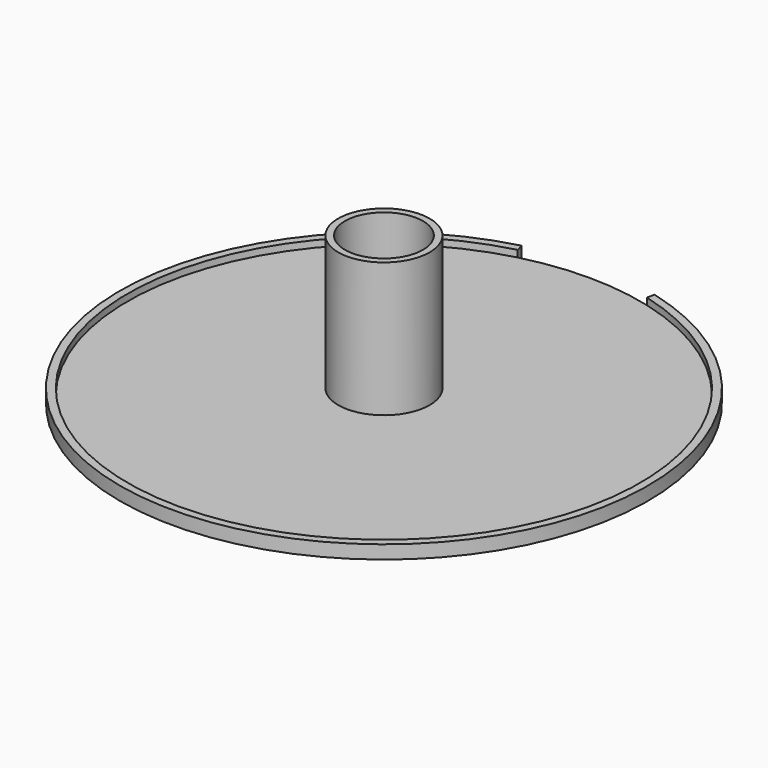
from build123d import *

# Parameters (mm, degrees)
F0_R     = 8.636
F0_R_2   = 7.366
F1_DEPTH = 25.4
F2_R     = 49.8475
F2_R_2   = 8.636
F2_R_3   = 7.366
F3_DEPTH = 2.54
F4_R     = 48.387
F5_DEPTH = 1.27
F7_DEPTH = 25.4


# Not quite as in the source:
# - a feature names something its author has since deleted; it is built from what else it names


with BuildPart() as f1:
    # F0 (on Top) → F1 (new body)
    with BuildSketch(Plane.XY):
        Circle(F0_R)
        Circle(F0_R_2, mode=Mode.SUBTRACT)
    extrude(amount=-F1_DEPTH)


with BuildPart() as f3:
    # F2 (on face) → F3 (new body)
    with BuildSketch(Plane(origin=(0, 0, -25.4), x_dir=(1, 0, 0), z_dir=(0, 0, -1))):
        Circle(F2_R)
        Circle(F2_R_2, mode=Mode.SUBTRACT)
        Circle(F2_R_2)
        Circle(F2_R_3, mode=Mode.SUBTRACT)
        Circle(F2_R_3)
    extrude(amount=F3_DEPTH)

    # F4 (on face) → F5 (cut)
    with BuildSketch(Plane.XY.offset(-25.4)):
        Circle(F4_R)
    extrude(amount=-F5_DEPTH, mode=Mode.SUBTRACT)

    # F6 (on face) → F7 (cut)
    with BuildSketch(Plane.XY.offset(-25.4)):
        with BuildLine():
            ThreePointArc((-12.192, 46.8258145151), (-6.1457742417, 47.9951167096), (0, 48.387))
            ThreePointArc((0, 48.387), (6.1457742417, 47.9951167096), (12.192, 46.8258145151))
            Line((12.192, 46.8258145151), (12.4823854572, 48.2593339112))
            ThreePointArc((12.4823854572, 48.2593339112), (-0.0443521709, 49.8474802687), (-12.5682438369, 48.2370449251))
            Line((-12.5682438369, 48.2370449251), (-12.192, 46.8258145151))
        make_face()
    extrude(amount=-F7_DEPTH, mode=Mode.SUBTRACT)


solid = Compound([f1.part, f3.part])
